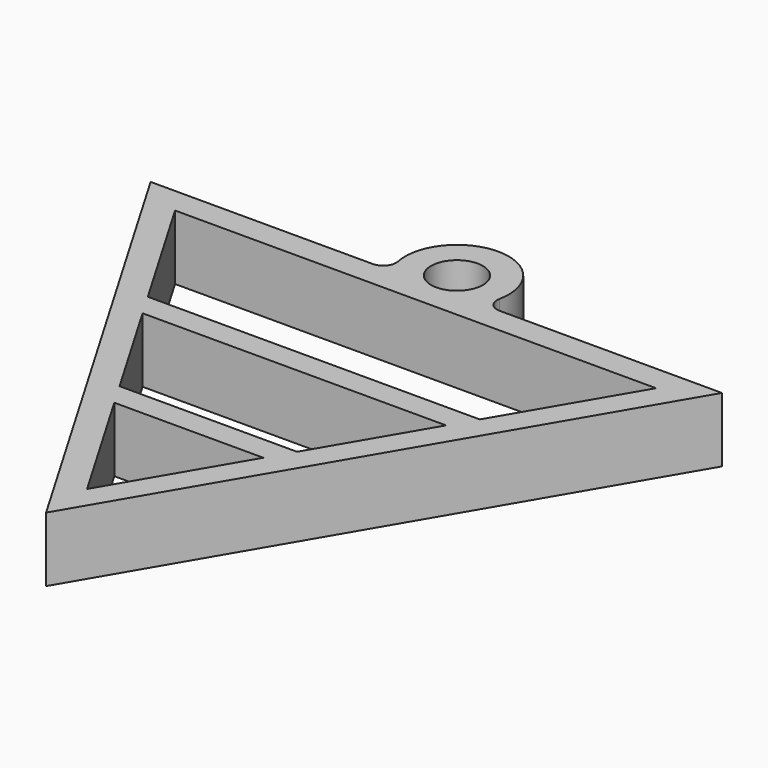
from build123d import *

# Parameters (mm, degrees)
F0_R         = 2
F1_DEPTH     = 2.5
F2_TEXT_SIZE = 5.2386658444
F3_DEPTH     = 1


# Not quite as in the source:
# - Text() gives the source's letters only with a copy of the font that has no kerning and outlines rounded to 1/6400 em; it was checked with that copy


with BuildPart() as f1:
    # F0 (on Top) → F1 (new body, symmetric)
    with BuildSketch(Plane.XY):
        with BuildLine():
            Line((-12.6661981972, 14.0163746178), (9.4053749926, -23.6691481605))
            Line((9.4053749926, -23.6691481605), (31.4769481825, 14.0163746178))
            Line((31.4769481825, 14.0163746178), (14.3043544782, 14.0163746178))
            ThreePointArc((14.3043544782, 14.0163746178), (13.529757809, 14.3839190858), (13.3245585811, 15.2163746178))
            ThreePointArc((13.3245585811, 15.2163746178), (9.4053749926, 20.0163746178), (5.4861914042, 15.2163746178))
            ThreePointArc((5.4861914042, 15.2163746178), (5.2809921763, 14.3839190858), (4.5063955071, 14.0163746178))
            Line((4.5063955071, 14.0163746178), (-12.6661981972, 14.0163746178))
        make_face()
        Polygon((15.1620537036, -9.8826387551), (9.4053749926, -19.7117272764), (3.6486962817, -9.8826387551), (9.4053749926, -9.8826387551), align=None, mode=Mode.SUBTRACT)
        Polygon((9.4053749926, -8.001949949), (2.5472186433, -8.001949949), (-2.3189128304, 0.3065972904), (9.4053749926, 0.3065972904), (21.1296628157, 0.3065972904), (16.2635313419, -8.001949949), align=None, mode=Mode.SUBTRACT)
        Polygon((-3.4203904688, 2.1872860965), (-9.1770691797, 12.0163746178), (9.4053749926, 12.0163746178), (27.987819165, 12.0163746178), (22.2311404541, 2.1872860965), (9.4053749926, 2.1872860965), align=None, mode=Mode.SUBTRACT)
        with Locations((9.4053749926, 16.0163746178)):
            Circle(F0_R, mode=Mode.SUBTRACT)
    extrude(amount=F1_DEPTH, both=True)

    # F2 (on face) → F3 (cut)
    with BuildSketch(Plane(origin=(-3.3187325527, -1.9437079025, 0), x_dir=(0.5053796547, -0.8628970996, 0), z_dir=(-0.8628970996, -0.5053796547, 0))):
        with Locations((-9.1084999602, -1.885919704)):
            Text('RESISTOR', F2_TEXT_SIZE, font='Open Sans', font_style=FontStyle.BOLD, text_align=(TextAlign.LEFT, TextAlign.BOTTOM))
    extrude(amount=-F3_DEPTH, mode=Mode.SUBTRACT)


solid = f1.part
